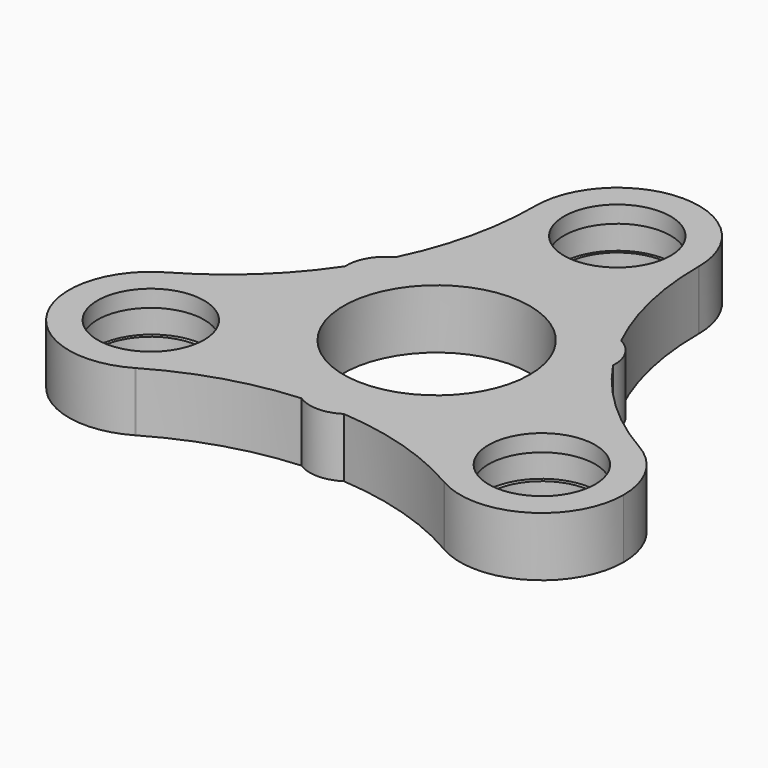
from build123d import *

# Parameters (mm, degrees)
F0_R     = 6.2993
F0_R_2   = 11
F1_DEPTH = 7
F4_R     = 6.6710532067
F5_DEPTH = 3


# Not quite as in the source:
# - ends of sketch curves that miss each other by under 0.0002 mm in the source are joined
# - a feature names something its author has since deleted; it is built from what else it names


with BuildPart() as f1:
    # F0 (on Top) → F1 (new body)
    with BuildSketch(Plane.XY):
        with BuildLine():
            ThreePointArc((9.6625090534, -0.0929069647), (9.6627025372, -0.0464533389), (9.6629557026, 0))
            ThreePointArc((9.6629557026, 0), (0, 9.6629557026), (-9.6629557026, 0))
            ThreePointArc((-9.6629557026, 0), (-9.662702535, -0.0464535369), (-9.6625090496, -0.0929073607))
            ThreePointArc((-9.6625090496, -0.0929073607), (1.98e-07, -9.6629557026), (9.6625090534, -0.0929069647))
        make_face()
        Circle(F0_R, mode=Mode.SUBTRACT)
        with BuildLine():
            ThreePointArc((-13.4378241011, -40.0117243144), (-18.2291272521, -31.6666830127), (-27.8515741938, -31.5972923328))
            ThreePointArc((-27.8515741938, -31.5972923328), (-27.8919011281, -31.6203516814), (-27.9322576549, -31.6433592003))
            ThreePointArc((-27.9322576549, -31.6433592003), (-31.4691449177, -44.8432021657), (-18.2693019524, -48.3800894285))
            ThreePointArc((-18.2693019524, -48.3800894285), (-18.2291987635, -48.3566435113), (-18.1890654853, -48.3332491365))
            ThreePointArc((-18.1890654853, -48.3332491365), (-14.7092843829, -44.8029159735), (-13.4378241011, -40.0117243144))
        make_face()
        with Locations((-23.1007798037, -40.0117243144)):
            Circle(F0_R, mode=Mode.SUBTRACT)
        with BuildLine():
            ThreePointArc((27.9322576549, -31.6433592003), (27.8919013007, -31.6203517785), (27.8515745387, -31.5972925275))
            ThreePointArc((27.8515745387, -31.5972925275), (14.7324146896, -35.1802464631), (18.1890654853, -48.3332491365))
            ThreePointArc((18.1890654853, -48.3332491365), (18.2291987635, -48.3566435113), (18.2693019524, -48.3800894285))
            ThreePointArc((18.2693019524, -48.3800894285), (27.9322576549, -48.3800894285), (32.7637355062, -40.0117243144))
            ThreePointArc((32.7637355062, -40.0117243144), (31.4691449177, -35.1802464631), (27.9322576549, -31.6433592003))
        make_face()
        with Locations((23.1007798037, -40.0117243144)):
            Circle(F0_R, mode=Mode.SUBTRACT)
        with BuildLine():
            ThreePointArc((13.3320983645, -16.0921664972), (10.5773906807, -8.3035279339), (9.6625090534, -0.0929069647))
            ThreePointArc((9.6625090534, -0.0929069647), (1.98e-07, -9.6629557026), (-9.6625090496, -0.0929073607))
            ThreePointArc((-9.6625090496, -0.0929073607), (-10.5773905595, -8.3035281796), (-13.3320981392, -16.0921666073))
            ThreePointArc((-13.3320981392, -16.0921666073), (-14.506503102, -18.2991494053), (-15.8306037894, -20.4197053365))
            ThreePointArc((-15.8306037894, -20.4197053365), (-21.1984087389, -26.6996712943), (-27.8515741938, -31.5972923328))
            ThreePointArc((-27.8515741938, -31.5972923328), (-18.2291272521, -31.6666830127), (-13.4378241011, -40.0117243144))
            ThreePointArc((-13.4378241011, -40.0117243144), (-14.7092843829, -44.8029159735), (-18.1890654853, -48.3332491365))
            ThreePointArc((-18.1890654853, -48.3332491365), (-10.6210183315, -45.0202493827), (-2.4985056329, -43.5115769352))
            ThreePointArc((-2.4985056329, -43.5115769352), (0, -43.4251500733), (2.4985056329, -43.5115769352))
            ThreePointArc((2.4985056329, -43.5115769352), (10.6210183315, -45.0202493827), (18.1890654853, -48.3332491365))
            ThreePointArc((18.1890654853, -48.3332491365), (14.7324146896, -35.1802464631), (27.8515745387, -31.5972925275))
            ThreePointArc((27.8515745387, -31.5972925275), (21.1984090122, -26.6996713122), (15.8306039974, -20.4197051964))
            ThreePointArc((15.8306039974, -20.4197051964), (14.506503323, -18.2991492777), (13.3320983645, -16.0921664972))
        make_face()
        with Locations((0, -26.6744828763)):
            Circle(F0_R_2, mode=Mode.SUBTRACT)
        with BuildLine():
            ThreePointArc((15.8306039974, -20.4197051964), (15.223256939, -17.8853313846), (13.3320983645, -16.0921664972))
            ThreePointArc((13.3320983645, -16.0921664972), (14.506503323, -18.2991492777), (15.8306039974, -20.4197051964))
        make_face()
        with BuildLine():
            ThreePointArc((-15.8306037894, -20.4197053365), (-14.506503102, -18.2991494053), (-13.3320981392, -16.0921666073))
            ThreePointArc((-13.3320981392, -16.0921666073), (-15.223256939, -17.8853313846), (-15.8306037894, -20.4197053365))
        make_face()
        with BuildLine():
            ThreePointArc((-2.4985056329, -43.5115769352), (0, -44.2527858596), (2.4985056329, -43.5115769352))
            ThreePointArc((2.4985056329, -43.5115769352), (0, -43.4251500733), (-2.4985056329, -43.5115769352))
        make_face()
    extrude(amount=F1_DEPTH)

    # F4 (on line) → F5 (cut)
    with BuildSketch(Plane.XY.offset(2)):
        Circle(F4_R)
        with Locations((-23.0745827089, -39.8926408961)):
            Circle(F4_R)
        with Locations((23.0107490857, -39.9294952557)):
            Circle(F4_R)
    extrude(amount=F5_DEPTH, mode=Mode.SUBTRACT)


solid = f1.part
